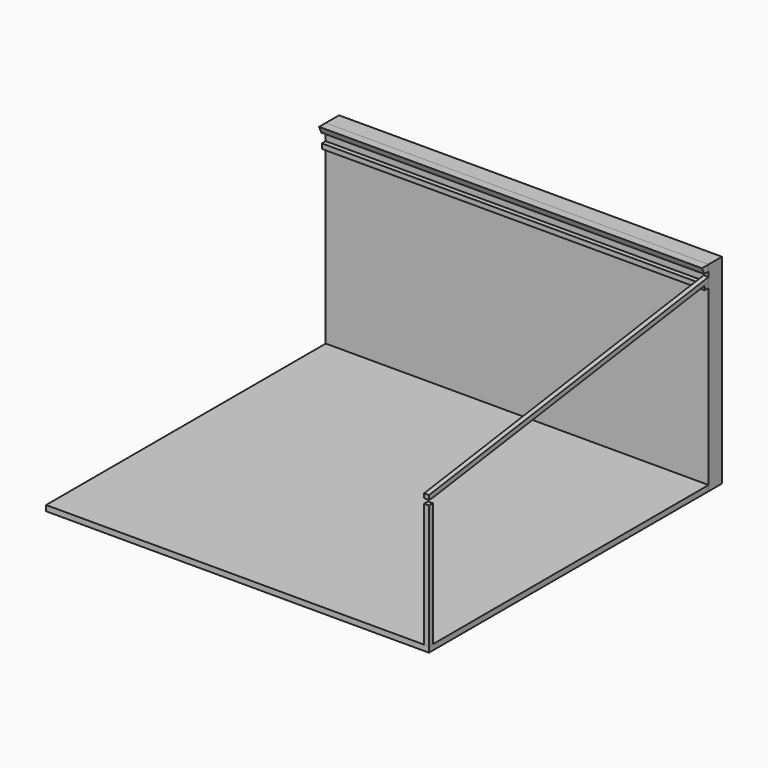
from build123d import *

# Parameters (mm, degrees)
F2_DEPTH  = 304.8
F4_DEPTH  = 7010.4
F1_E1_W   = 3505.2
F1_E1_H   = 6400.8
F1_E0_W   = 3505.2
F1_E0_H   = 6400.8
F5_DEPTH  = 101.6
F7_DEPTH  = 88.9
F8_DEPTH  = 88.9
F9_DEPTH  = 7010.4
F11_DEPTH = 88.9


with BuildPart() as f2:
    # F0 (on Front) → F2 (new body)
    with BuildSketch(Plane.XZ):
        Polygon((-3505.2, 0), (0, 0), (3505.2, 0), (3505.2, 3657.6), (-3505.2, 3657.6), align=None)
    extrude(amount=-F2_DEPTH)


with BuildPart() as f4:
    # F3 (on face) → F4 (new body)
    with BuildSketch(Plane.YZ.offset(3505.2)):
        Polygon((0, 3543.3), (0, 3657.6), (-152.4, 3657.6), (-101.6, 3543.3), align=None)
    extrude(amount=-F4_DEPTH)


with BuildPart() as f5:
    # F1_E1 (on explicit) + F1_E0 (on explicit) → F5 (new body)
    with BuildSketch(Plane(origin=(0, 0, 0), x_dir=(-1, 0, 0), z_dir=(0, 0, 1))):
        with Locations((1752.6, 3200.4)):
            Rectangle(F1_E1_W, F1_E1_H)
    with BuildSketch(Plane(origin=(0, 0, 0), x_dir=(1, 0, 0), z_dir=(0, 0, -1))):
        with Locations((1752.6, 3200.4)):
            Rectangle(F1_E0_W, F1_E0_H)
    extrude(amount=F5_DEPTH, dir=(0, 0, 1))


with BuildPart() as f7:
    # F6 (on face) → F7 (new body)
    with BuildSketch(Plane.YZ.offset(3505.2)):
        Polygon((-6400.8, 101.6), (-6311.9, 101.6), (-6311.9, 2462.8974387893), (-6400.8, 2450.1974387893), align=None)
    extrude(amount=-F7_DEPTH)


with BuildPart() as f8:
    # F6 (on face) → F8 (new body)
    with BuildSketch(Plane.YZ.offset(3505.2)):
        Polygon((-88.9, 3364.5974387893), (0, 3364.5974387893), (0, 3454.4), (-6400.8, 2540), (-6400.8, 2450.1974387893), (-6311.9, 2462.8974387893), (-88.9, 3351.8974387893), align=None)
    extrude(amount=-F8_DEPTH)


with BuildPart() as f9:
    # F6 (on face) → F9 (new body)
    with BuildSketch(Plane.YZ.offset(3505.2)):
        Polygon((-88.9, 3275.6974387893), (0, 3275.6974387893), (0, 3364.5974387893), (-88.9, 3351.8974387893), align=None)
        Polygon((-88.9, 3351.8974387893), (0, 3364.5974387893), (-88.9, 3364.5974387893), align=None)
    extrude(amount=-F9_DEPTH)


with BuildPart() as f11_tool:
    # F10 (on face) → F11 (new body)
    with BuildSketch(Plane.YZ.offset(3505.2)):
        Polygon((-6311.9, 2373.9974387893), (-6311.9, 2462.8974387893), (-6400.8, 2450.1974387893), (-6400.8, 2373.9974387893), align=None)
        Polygon((-6400.8, 2450.1974387893), (-6311.9, 2462.8974387893), (-6400.8, 2462.8974387893), align=None)
    extrude(amount=-F11_DEPTH)


with BuildPart() as f7_1:
    add(f7.part)

    # F11: cut by f11_tool
    add(f11_tool.part, mode=Mode.SUBTRACT)


with BuildPart() as f8_1:
    add(f8.part)

    # F11: cut by f11_tool
    add(f11_tool.part, mode=Mode.SUBTRACT)


solid = Compound([f2.part, f4.part, f5.part, f9.part, f7_1.part, f8_1.part])
